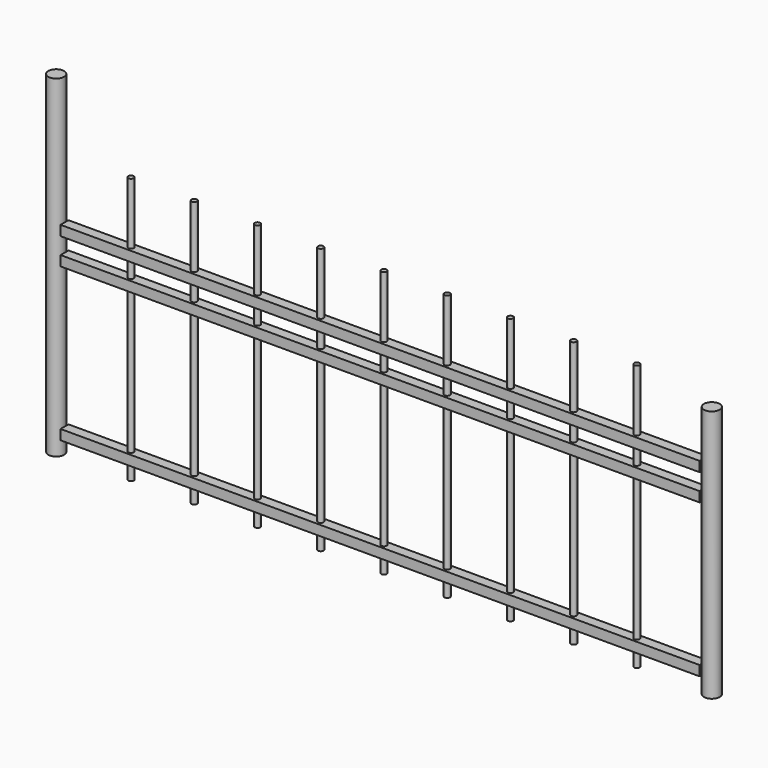
from build123d import *

# Parameters (mm, degrees)
F7_R           = 10.668
F9_DEPTH       = 1016
F10_DEPTH      = 1016
F11_DEPTH      = 1016
F8_W           = 38.1
F8_H           = 38.1
F12_DEPTH      = 2184.4
F12_DEPTH_BACK = 254
F7_R_2         = 30.1625
F13_DEPTH      = 1270
F14_DEPTH      = 965.2


# Not quite as in the source:
# - a variable given as a bare number and used for a length is read in inches; the dataset says mm whatever the document's units were
# - a feature names something its author has since deleted; it is built from what else it names


with BuildPart() as f9:
    # F7 (on Top) → F9 (new body)
    with BuildSketch(Plane.XY):
        Circle(F7_R)
    extrude(amount=F9_DEPTH)



with BuildPart() as f9b:
    # F7 (on Top) → F9, piece 2 (new body)
    with BuildSketch(Plane.XY):
        with Locations((965.2, 0)):
            Circle(F7_R)
    extrude(amount=F9_DEPTH)


with BuildPart() as f9c:
    # F7 (on Top) → F9, piece 3 (new body)
    with BuildSketch(Plane.XY):
        with Locations((1930.4, 0)):
            Circle(F7_R)
    extrude(amount=F9_DEPTH)


with BuildPart() as f10:
    # F7 (on Top) → F10 (new body)
    with BuildSketch(Plane.XY):
        with Locations((241.3, 0)):
            Circle(F7_R)
    extrude(amount=F10_DEPTH)


with BuildPart() as f10b:
    # F7 (on Top) → F10, piece 2 (new body)
    with BuildSketch(Plane.XY):
        with Locations((723.9, 0)):
            Circle(F7_R)
    extrude(amount=F10_DEPTH)


with BuildPart() as f10c:
    # F7 (on Top) → F10, piece 3 (new body)
    with BuildSketch(Plane.XY):
        with Locations((1206.5, 0)):
            Circle(F7_R)
    extrude(amount=F10_DEPTH)


with BuildPart() as f10d:
    # F7 (on Top) → F10, piece 4 (new body)
    with BuildSketch(Plane.XY):
        with Locations((1689.1, 0)):
            Circle(F7_R)
    extrude(amount=F10_DEPTH)


with BuildPart() as f11:
    # F7 (on Top) → F11 (new body)
    with BuildSketch(Plane.XY):
        with Locations((482.6, 0)):
            Circle(F7_R)
    extrude(amount=F11_DEPTH)


with BuildPart() as f11b:
    # F7 (on Top) → F11, piece 2 (new body)
    with BuildSketch(Plane.XY):
        with Locations((1447.8, 0)):
            Circle(F7_R)
    extrude(amount=F11_DEPTH)


with BuildPart() as f9_1:
    add(f9.part)

    add(f9b.part)  # F12 merges F9b

    add(f9c.part)  # F12 merges F9c

    add(f10.part)  # F12 merges F10

    add(f10b.part)  # F12 merges F10b

    add(f10c.part)  # F12 merges F10c

    add(f10d.part)  # F12 merges F10d

    add(f11.part)  # F12 merges F11

    add(f11b.part)  # F12 merges F11b
    # F8 (on Right) → F12 (join, two sides)
    with BuildSketch(Plane.YZ) as f12_sk:
        with Locations((0, 762)):
            Rectangle(F8_W, F8_H)
        with Locations((0, 660.4)):
            Rectangle(F8_W, F8_H)
        with Locations((0, 76.2)):
            Rectangle(F8_W, F8_H)
    extrude(amount=F12_DEPTH)
    extrude(f12_sk.sketch, amount=-F12_DEPTH_BACK)


with BuildPart() as f13:
    # F7 (on Top) → F13 (new body)
    with BuildSketch(Plane.XY):
        with Locations((-285.75, 0)):
            Circle(F7_R_2)
    extrude(amount=F13_DEPTH)


with BuildPart() as f14:
    # F7 (on Top) → F14 (new body)
    with BuildSketch(Plane.XY):
        with Locations((2216.15, 0)):
            Circle(F7_R_2)
    extrude(amount=F14_DEPTH)


solid = Compound([f9_1.part, f13.part, f14.part])
